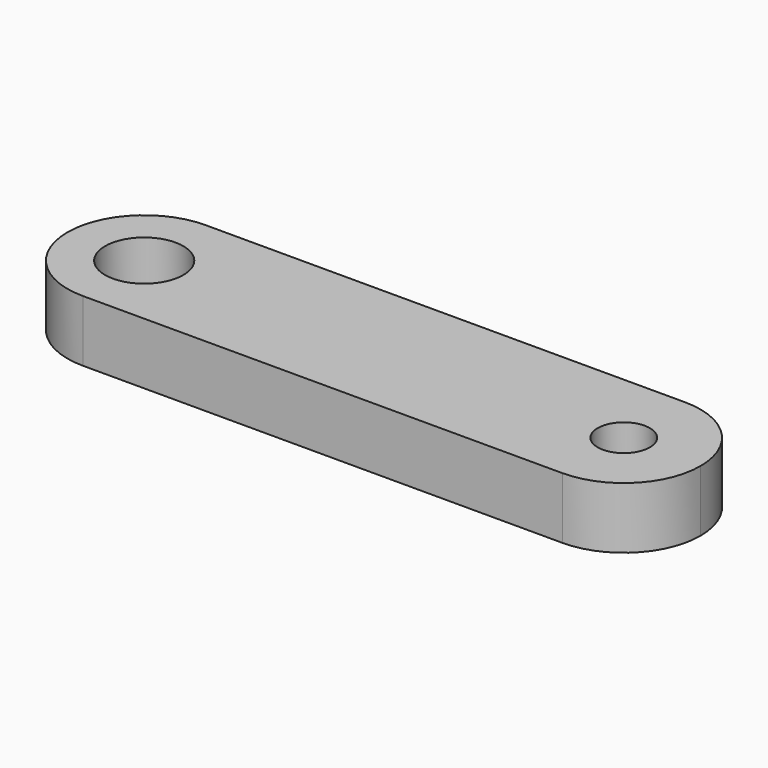
from build123d import *

# Parameters (mm, degrees)
F0_W     = 82.5
F0_H     = 20
F1_DEPTH = 8
F2_D     = 10.2
F3_D     = 6.8
F4_R     = 9.99999


# Not quite as in the source:
# - a fillet or chamfer is up to 0.001 mm smaller than in the source, because OpenCascade refuses the exact size


with BuildPart() as f1:
    # F0 (on Top) → F1 (new body)
    with BuildSketch(Plane.XY):
        Rectangle(F0_W, F0_H)
    extrude(amount=-F1_DEPTH)

    # F2 (through all)
    with Locations(Plane.XY):
        with Locations((-31.25, 0)):
            Hole(F2_D / 2)

    # F3 (through all)
    with Locations(Plane.XY):
        with Locations((31.25, 0)):
            Hole(F3_D / 2)

    # F4 (radius 10 in the source; OpenCascade refuses exactly that, so slightly less here)
    f4_edges = [f1.edges().sort_by_distance(p)[0] for p in [
        (41.25, 10, -4),
        (41.25, -10, -4),
        (-41.25, 10, -4),
        (-41.25, -10, -4),
    ]]
    fillet(f4_edges, radius=F4_R)


solid = f1.part
